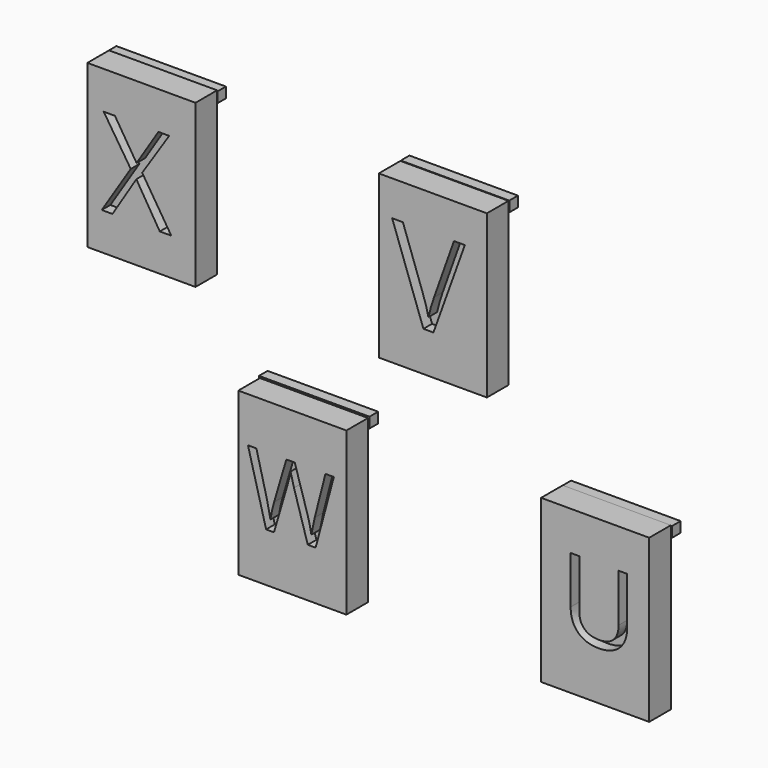
from build123d import *

# Parameters (mm, degrees)
F0_W           = 25.4
F0_H           = 38.1
F1_DEPTH       = 6.35
F2_R           = 3.81
F3_DEPTH       = 2.54
F5_TEXT_SIZE   = 24.2855962521
F5_TEXT_SIZE_2 = 28.7011576196
F5_TEXT_SIZE_3 = 22.4457769137
F5_TEXT_SIZE_4 = 28.7011615001
F6_DEPTH       = 25.4
F7_W           = 25.730624795
F7_H           = 2.4505369365
F8_DEPTH       = 2.54
F7_W_2         = 25.4855751991
F7_W_3         = 25.7306285203
F7_W_4         = 25.9756827727
F7_H_2         = 2.4505350739


# Not quite as in the source:
# - Text() gives the source's letters only with a copy of the font that has no kerning and outlines rounded to 1/6400 em; it was checked with that copy


with BuildPart() as f1:
    # F0 (on Front) → F1 (new body)
    with BuildSketch(Plane.XZ):
        with Locations((-46.0602159804, 19.2970331914)):
            Rectangle(F0_W, F0_H)
    extrude(amount=F1_DEPTH)

    # F2 (on Front) → F3, piece 2 (join)
    with BuildSketch(Plane.XZ):
        with Locations((-40.9802159804, 28.1870331914)):
            Circle(F2_R)
        with Locations((-51.1402159804, 28.1870331914)):
            Circle(F2_R)
        with Locations((-51.1402159804, 7.8670331914)):
            Circle(F2_R)
        with Locations((-40.9802159804, 7.8670331914)):
            Circle(F2_R)
    extrude(amount=-F3_DEPTH)


with BuildPart() as f1b:
    # F0 (on Front) → F1, piece 2 (new body)
    with BuildSketch(Plane.XZ):
        with Locations((-10.603061258, -36.9614025138)):
            Rectangle(F0_W, F0_H)
    extrude(amount=F1_DEPTH)

    # F2 (on Front) → F3, piece 4 (join)
    with BuildSketch(Plane.XZ):
        with Locations((-5.523061258, -38.2314025138)):
            Circle(F2_R)
        with Locations((-15.683061258, -28.0714025138)):
            Circle(F2_R)
        with Locations((-15.683061258, -48.3914025138)):
            Circle(F2_R)
        with Locations((-15.683061258, -38.2314025138)):
            Circle(F2_R)
    extrude(amount=-F3_DEPTH)


with BuildPart() as f1c:
    # F0 (on Front) → F1, piece 3 (new body)
    with BuildSketch(Plane.XZ):
        with Locations((60.5514380593, -36.0065931796)):
            Rectangle(F0_W, F0_H)
    extrude(amount=F1_DEPTH)

    # F2 (on Front) → F3, piece 3 (join)
    with BuildSketch(Plane.XZ):
        with Locations((65.6314380593, -27.1165931796)):
            Circle(F2_R)
        with Locations((65.6314380593, -47.4365931796)):
            Circle(F2_R)
        with Locations((55.4714380593, -47.4365931796)):
            Circle(F2_R)
    extrude(amount=-F3_DEPTH)


with BuildPart() as f1d:
    # F0 (on Front) → F1, piece 4 (new body)
    with BuildSketch(Plane.XZ):
        with Locations((22.4085926682, 18.6961098781)):
            Rectangle(F0_W, F0_H)
    extrude(amount=F1_DEPTH)

    # F2 (on Front) → F3 (join)
    with BuildSketch(Plane.XZ):
        with Locations((27.4885926682, 7.2661098781)):
            Circle(F2_R)
        with Locations((27.4885926682, 17.4261098781)):
            Circle(F2_R)
        with Locations((27.4885926682, 27.5861098781)):
            Circle(F2_R)
        with Locations((17.3285926682, 7.2661098781)):
            Circle(F2_R)
    extrude(amount=-F3_DEPTH)


with BuildPart() as f6_tool:
    # F5 (on offset) → F6 (new body)
    with BuildSketch(Plane.XZ.offset(3.81)):
        with Locations((52.5903739035, -43.4491387568)):
            Text('U', F5_TEXT_SIZE, font='Open Sans', text_align=(TextAlign.LEFT, TextAlign.BOTTOM))
        with Locations((12.8502957523, 9.0077463537)):
            Text('V', F5_TEXT_SIZE_2, font='Open Sans', text_align=(TextAlign.LEFT, TextAlign.BOTTOM))
        with Locations((-21.3261516765, -44.5088744164)):
            Text('W', F5_TEXT_SIZE_3, font='Open Sans', text_align=(TextAlign.LEFT, TextAlign.BOTTOM))
        with Locations((-55.502615869, 9.0077491477)):
            Text('X', F5_TEXT_SIZE_4, font='Open Sans', text_align=(TextAlign.LEFT, TextAlign.BOTTOM))
    extrude(amount=F6_DEPTH)


with BuildPart() as f1_1:
    add(f1.part)

    # F6: cut by f6_tool
    add(f6_tool.part, mode=Mode.SUBTRACT)

    # F7 (on Front) → F8, piece 3 (join)
    with BuildSketch(Plane.XZ):
        with Locations((-46.1926031858, 36.8805658072)):
            Rectangle(F7_W_3, F7_H)
    extrude(amount=-F8_DEPTH)


with BuildPart() as f1b_1:
    add(f1b.part)

    # F6: cut by f6_tool
    add(f6_tool.part, mode=Mode.SUBTRACT)

    # F7 (on Front) → F8, piece 4 (join)
    with BuildSketch(Plane.XZ):
        with Locations((-10.5373053811, -18.7466004863)):
            Rectangle(F7_W_4, F7_H_2)
    extrude(amount=-F8_DEPTH)


with BuildPart() as f1c_1:
    add(f1c.part)

    # F6: cut by f6_tool
    add(f6_tool.part, mode=Mode.SUBTRACT)

    # F7 (on Front) → F8 (join)
    with BuildSketch(Plane.XZ):
        with Locations((60.6507658958, -18.2564929128)):
            Rectangle(F7_W, F7_H)
    extrude(amount=-F8_DEPTH)


with BuildPart() as f1d_1:
    add(f1d.part)

    # F6: cut by f6_tool
    add(f6_tool.part, mode=Mode.SUBTRACT)

    # F7 (on Front) → F8, piece 2 (join)
    with BuildSketch(Plane.XZ):
        with Locations((22.5449316204, 36.6355124861)):
            Rectangle(F7_W_2, F7_H)
    extrude(amount=-F8_DEPTH)


solid = Compound([f1_1.part, f1b_1.part, f1c_1.part, f1d_1.part])
